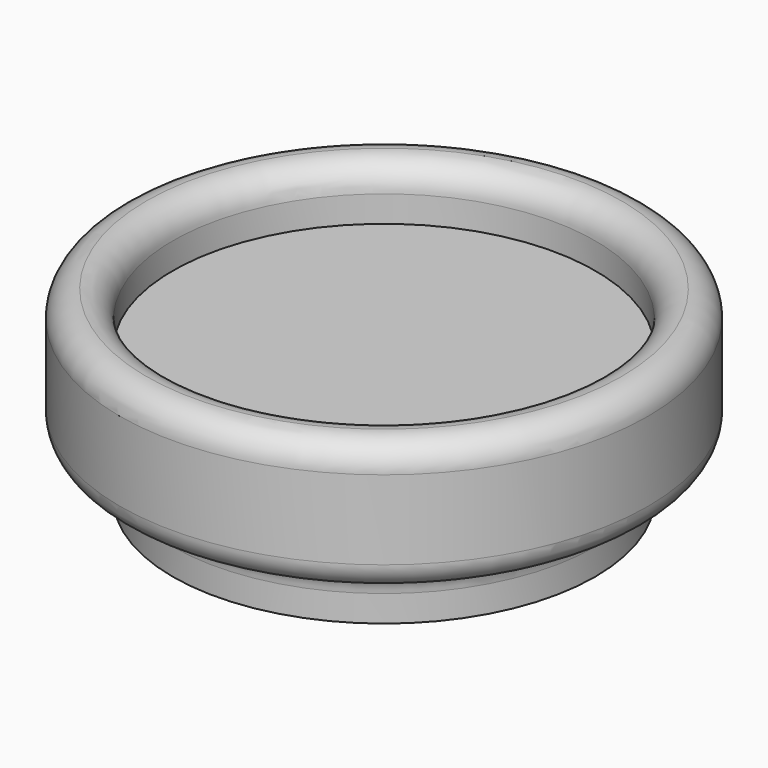
from build123d import *

# Parameters (mm, degrees)
F0_R     = 10
F1_DEPTH = 5
F2_R     = 8
F3_DEPTH = 2
F4_R     = 8
F5_DEPTH = 2
F6_R     = 0.99999


# Not quite as in the source:
# - a fillet or chamfer is up to 0.001 mm smaller than in the source, because OpenCascade refuses the exact size


with BuildPart() as f1:
    # F0 (on Top) → F1 (new body)
    with BuildSketch(Plane.XY):
        Circle(F0_R)
    extrude(amount=F1_DEPTH)

    # F2 (on face) → F3 (join)
    with BuildSketch(Plane(origin=(0, 0, 0), x_dir=(1, 0, 0), z_dir=(0, 0, -1))):
        Circle(F2_R)
    extrude(amount=F3_DEPTH)

    # F4 (on face) → F5 (cut)
    with BuildSketch(Plane.XY.offset(5)):
        Circle(F4_R)
    extrude(amount=-F5_DEPTH, mode=Mode.SUBTRACT)

    # F6 (radius 1 in the source; OpenCascade refuses exactly that, so slightly less here)
    f6_edges = [f1.edges().sort_by_distance(p)[0] for p in [
        (-8, 0, 0),
        (-10, 0, 0),
        (-10, 0, 5),
        (-8, 0, 5),
    ]]
    fillet(f6_edges, radius=F6_R)


solid = f1.part
